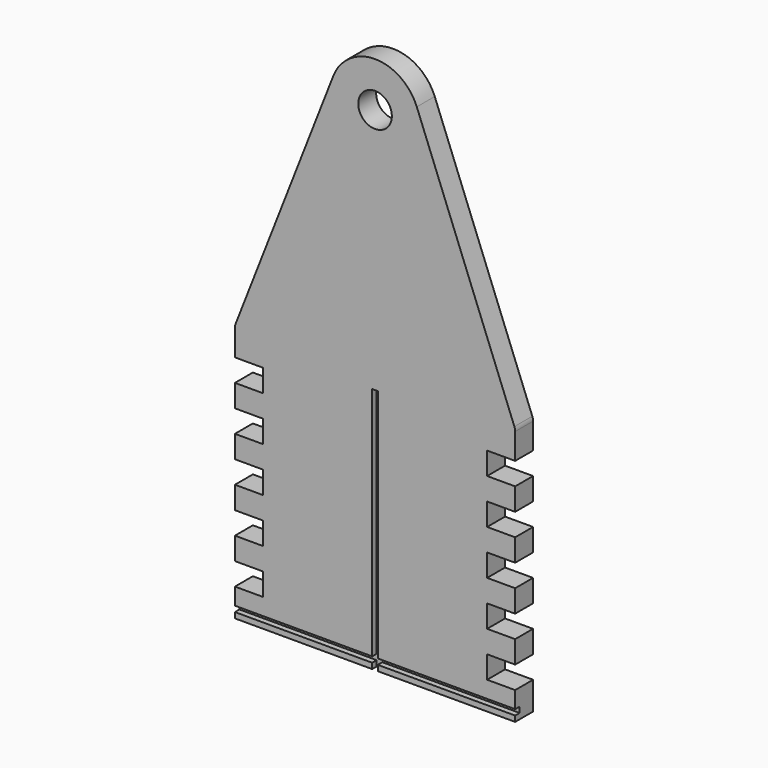
from build123d import *

# Parameters (mm, degrees)
F1_DEPTH = 9.525
F0_W     = 77.7875
F0_H     = 3.175
F0_W_2   = 77.8286574921
F0_R     = 9.525
F2_DEPTH = 12.7


with BuildPart() as f1:
    # F0 (on Front) → F1 (new body)
    with BuildSketch(Plane.XZ):
        Polygon((-1.5875, -69.85), (-1.5875, -73.025), (1.5463425079, -73.025), (1.5463425079, -69.85), (79.375, -69.85), (79.375, -66.675), (1.5875, -66.675), (1.5875, 66.675), (-1.5875, 66.675), (-1.5875, -66.675), (-79.375, -66.675), (-79.375, -69.85), align=None)
    extrude(amount=F1_DEPTH)

    # F0 (on Front) → F2 (join)
    with BuildSketch(Plane.XZ):
        with Locations((-40.48125, -71.4375)):
            Rectangle(F0_W, F0_H)
        with Locations((40.460671254, -71.4375)):
            Rectangle(F0_W_2, F0_H)
        with BuildLine():
            Line((-79.375, -57.15), (-79.375, -66.675))
            Line((-79.375, -66.675), (-1.5875, -66.675))
            Line((-1.5875, -66.675), (-1.5875, 66.675))
            Line((-1.5875, 66.675), (1.5875, 66.675))
            Line((1.5875, 66.675), (1.5875, -66.675))
            Line((1.5875, -66.675), (79.375, -66.675))
            Line((79.375, -66.675), (79.375, -57.15))
            Line((79.375, -57.15), (63.5, -57.15))
            Line((63.5, -57.15), (63.5, -44.45))
            Line((63.5, -44.45), (79.375, -44.45))
            Line((79.375, -44.45), (79.375, -31.75))
            Line((79.375, -31.75), (63.5, -31.75))
            Line((63.5, -31.75), (63.5, -19.05))
            Line((63.5, -19.05), (79.375, -19.05))
            Line((79.375, -19.05), (79.375, -6.35))
            Line((79.375, -6.35), (63.5, -6.35))
            Line((63.5, -6.35), (63.5, 6.35))
            Line((63.5, 6.35), (79.375, 6.35))
            Line((79.375, 6.35), (79.375, 19.05))
            Line((79.375, 19.05), (63.5, 19.05))
            Line((63.5, 19.05), (63.5, 31.75))
            Line((63.5, 31.75), (79.375, 31.75))
            Line((79.375, 31.75), (79.375, 44.45))
            Line((79.375, 44.45), (63.5, 44.45))
            Line((63.5, 44.45), (63.5, 57.15))
            Line((63.5, 57.15), (79.375, 57.15))
            Line((79.375, 57.15), (79.375, 71.8284572224))
            ThreePointArc((79.375, 71.8284572224), (79.2651824968, 73.0043068755), (78.9395283758, 74.1394860175))
            Line((78.9395283758, 74.1394860175), (23.6581135032, 215.6191151805))
            ThreePointArc((23.6581135032, 215.6191151805), (0, 231.775), (-23.6581135032, 215.6191151805))
            Line((-23.6581135032, 215.6191151805), (-78.9395283758, 74.1394860175))
            ThreePointArc((-78.9395283758, 74.1394860175), (-79.2651824968, 73.0043068755), (-79.375, 71.8284572224))
            Line((-79.375, 71.8284572224), (-79.375, 57.15))
            Line((-79.375, 57.15), (-63.5, 57.15))
            Line((-63.5, 57.15), (-63.5, 44.45))
            Line((-63.5, 44.45), (-79.375, 44.45))
            Line((-79.375, 44.45), (-79.375, 31.75))
            Line((-79.375, 31.75), (-63.5, 31.75))
            Line((-63.5, 31.75), (-63.5, 19.05))
            Line((-63.5, 19.05), (-79.375, 19.05))
            Line((-79.375, 19.05), (-79.375, 6.35))
            Line((-79.375, 6.35), (-63.5, 6.35))
            Line((-63.5, 6.35), (-63.5, -6.35))
            Line((-63.5, -6.35), (-79.375, -6.35))
            Line((-79.375, -6.35), (-79.375, -19.05))
            Line((-79.375, -19.05), (-63.5, -19.05))
            Line((-63.5, -19.05), (-63.5, -31.75))
            Line((-63.5, -31.75), (-79.375, -31.75))
            Line((-79.375, -31.75), (-79.375, -44.45))
            Line((-79.375, -44.45), (-63.5, -44.45))
            Line((-63.5, -44.45), (-63.5, -57.15))
            Line((-63.5, -57.15), (-79.375, -57.15))
        make_face()
        with Locations((0, 206.375)):
            Circle(F0_R, mode=Mode.SUBTRACT)
    extrude(amount=F2_DEPTH)


solid = f1.part
